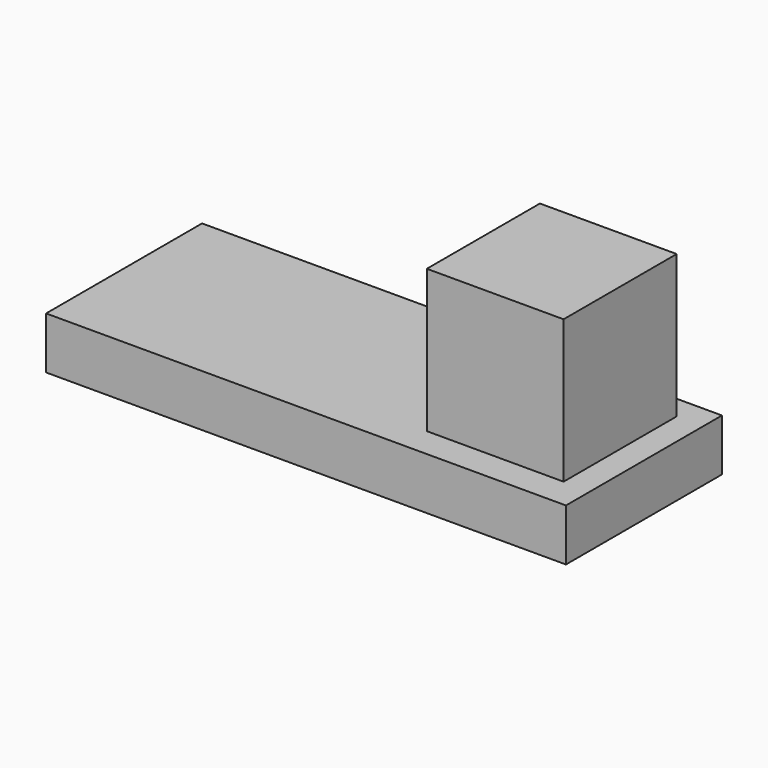
from build123d import *

# Parameters (mm, degrees)
F0_W     = 200
F0_H     = 20
F1_DEPTH = 75
F2_W     = 52.6148378849
F2_H     = 54.3804401532
F3_DEPTH = 55


# Not quite as in the source:
# - a feature names something its author has since deleted; it is built from what else it names


with BuildPart() as f1:
    # F0 (on Front) → F1 (new body)
    with BuildSketch(Plane.XZ):
        with Locations((39.6226420999, -12.8532575865)):
            Rectangle(F0_W, F0_H)
    extrude(amount=F1_DEPTH)

    # F2 (on face) → F3 (join)
    with BuildSketch(Plane.XY.offset(-2.8532575865)):
        with Locations((103.0974239111, -36.1731755547)):
            Rectangle(F2_W, F2_H)
    extrude(amount=F3_DEPTH)


solid = f1.part
